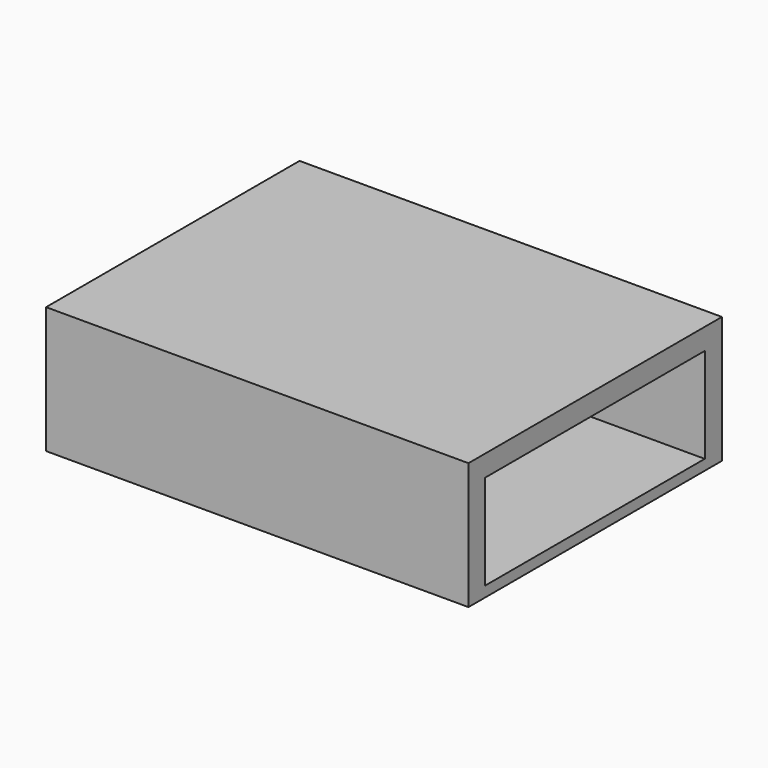
from build123d import *

# Parameters (mm, degrees)
F0_W     = 40
F0_H     = 30
F1_DEPTH = 12
F2_W     = 26
F2_H     = 9
F3_DEPTH = 38


# Not quite as in the source:
# - a feature names something its author has since deleted; it is built from what else it names


with BuildPart() as f1:
    # F0 (on Top) → F1 (new body)
    with BuildSketch(Plane.XY):
        with Locations((-1.1542569846, 12)):
            Rectangle(F0_W, F0_H)
    extrude(amount=F1_DEPTH)

    # F2 (on face) → F3 (cut)
    with BuildSketch(Plane.YZ.offset(18.8457430154)):
        with Locations((11.9680855733, 5.492781871)):
            Rectangle(F2_W, F2_H)
    extrude(amount=-F3_DEPTH, mode=Mode.SUBTRACT)


solid = f1.part
